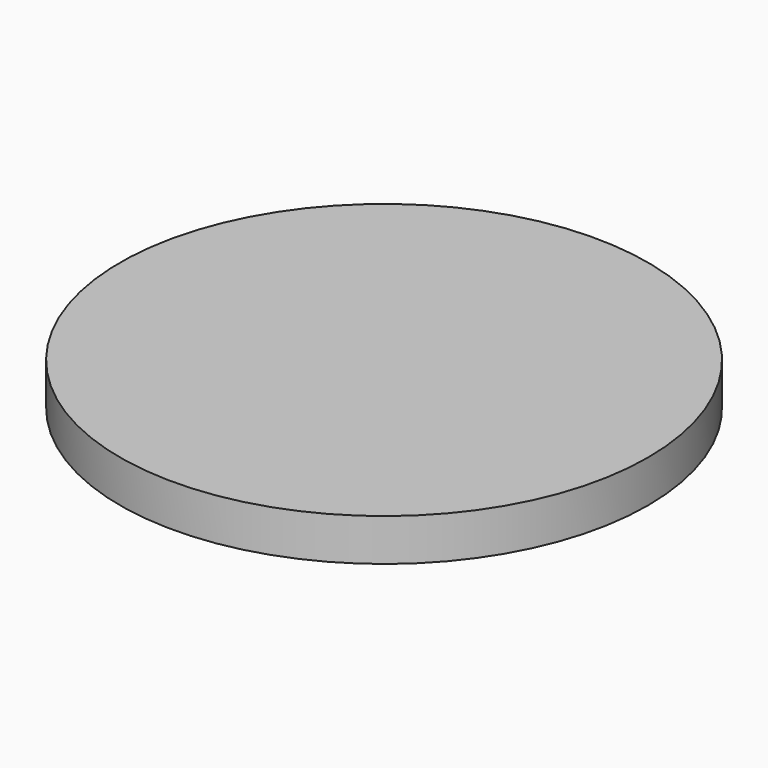
from build123d import *

# Parameters (mm, degrees)
F0_R     = 31.792212297
F1_DEPTH = 5.08


# Not quite as in the source:
# - the program builds the solid bodies; features that only make, move or delete a surface that nothing else refers to are left out


with BuildPart() as f1:
    # F0 (on Top) → F1 (new body)
    with BuildSketch(Plane.XY):
        Circle(F0_R)
    extrude(amount=F1_DEPTH)


solid = f1.part
